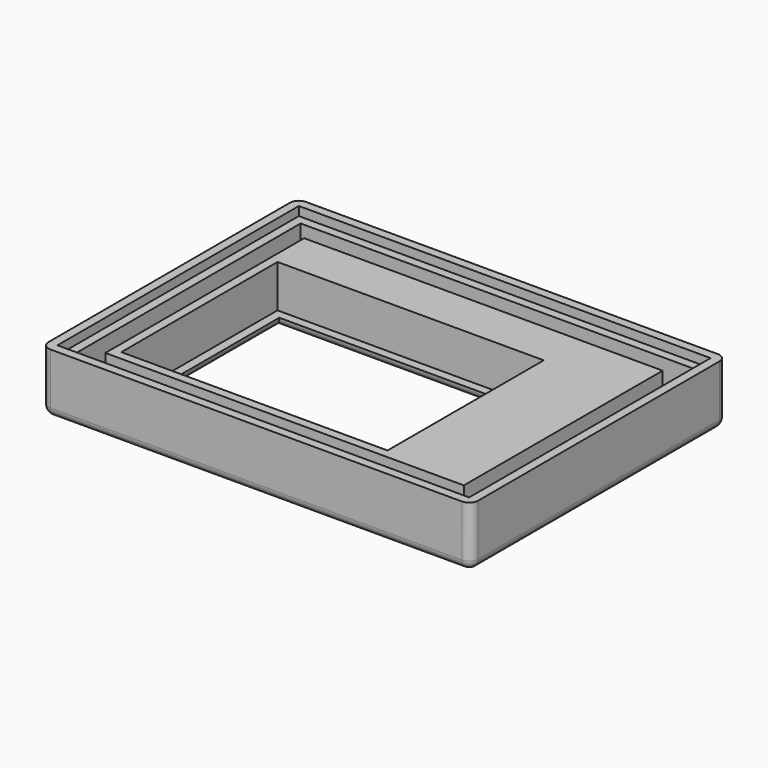
from build123d import *

# Parameters (mm, degrees)
F0_W     = 242
F0_H     = 180
F1_DEPTH = 34
F2_W     = 140
F2_H     = 100
F3_DEPTH = 34.001
F4_W     = 150
F4_H     = 110
F4_W_2   = 140
F4_H_2   = 100
F5_DEPTH = 29
F6_W     = 232
F6_H     = 170
F6_W_2   = 150
F6_H_2   = 110
F7_DEPTH = 5
F8_W     = 222
F8_H     = 160
F8_W_2   = 202
F8_H_2   = 140
F9_DEPTH = 20
F10_R    = 5
F11_R    = 4.99999


# Not quite as in the source:
# - a fillet or chamfer is up to 0.001 mm smaller than in the source, because OpenCascade refuses the exact size


with BuildPart() as f1:
    # F0 (on Top) → F1 (new body)
    with BuildSketch(Plane.XY):
        with Locations((121, 90)):
            Rectangle(F0_W, F0_H)
    extrude(amount=F1_DEPTH)

    # F2 (on face) → F3 (cut, through all)
    with BuildSketch(Plane.XY.offset(34)):
        with Locations((100, 80)):
            Rectangle(F2_W, F2_H)
    extrude(amount=-F3_DEPTH, mode=Mode.SUBTRACT)

    # F4 (on face) → F5 (cut)
    with BuildSketch(Plane.XY.offset(34)):
        with Locations((100, 80)):
            Rectangle(F4_W, F4_H)
        with Locations((100, 80)):
            Rectangle(F4_W_2, F4_H_2, mode=Mode.SUBTRACT)
    extrude(amount=-F5_DEPTH, mode=Mode.SUBTRACT)

    # F6 (on face) → F7 (cut)
    with BuildSketch(Plane.XY.offset(34)):
        with Locations((121, 90)):
            Rectangle(F6_W, F6_H)
        with Locations((100, 80)):
            Rectangle(F6_W_2, F6_H_2, mode=Mode.SUBTRACT)
    extrude(amount=-F7_DEPTH, mode=Mode.SUBTRACT)

    # F8 (on face) → F9 (cut)
    with BuildSketch(Plane.XY.offset(29)):
        with Locations((121, 90)):
            Rectangle(F8_W, F8_H)
        with Locations((121, 90)):
            Rectangle(F8_W_2, F8_H_2, mode=Mode.SUBTRACT)
    extrude(amount=-F9_DEPTH, mode=Mode.SUBTRACT)

    # F10
    f10_edges = [f1.edges().sort_by_distance(p)[0] for p in [
        (242, 0, 17),
        (242, 180, 17),
        (0, 180, 17),
        (0, 0, 17),
    ]]
    fillet(f10_edges, radius=F10_R)

    # F11 (radius 5 in the source; OpenCascade refuses exactly that, so slightly less here)
    f11_edges = [f1.edges().sort_by_distance(p)[0] for p in [
        (121, 0, 0),
        (170, 80, 0),
        (100, 30, 0),
        (30, 80, 0),
        (100, 130, 0),
    ]]
    fillet(f11_edges, radius=F11_R)


solid = f1.part
